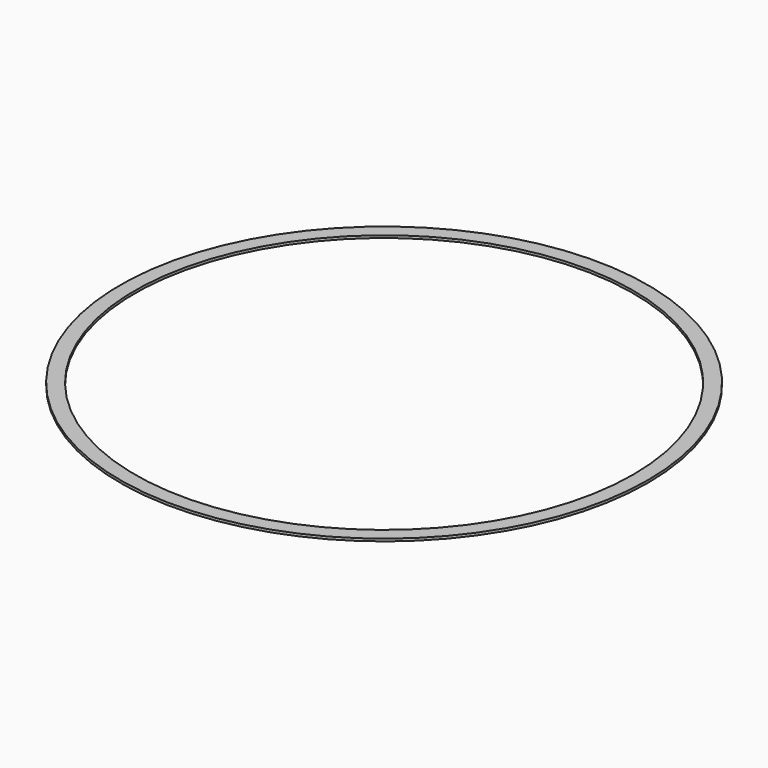
from build123d import *

# Parameters (mm, degrees)
F0_R     = 453.45858
F0_R_2   = 428.05858
F1_DEPTH = 4.2333333333


# Not quite as in the source:
# - a length typed as a fraction of an inch, garbled in the dataset ("3 / 203.2 mm" for 3/8 in), is restored


with BuildPart() as f1:
    # F0 (on Top) → F1 (new body)
    with BuildSketch(Plane.XY):
        Circle(F0_R)
        Circle(F0_R_2, mode=Mode.SUBTRACT)
    extrude(amount=F1_DEPTH)


solid = f1.part
